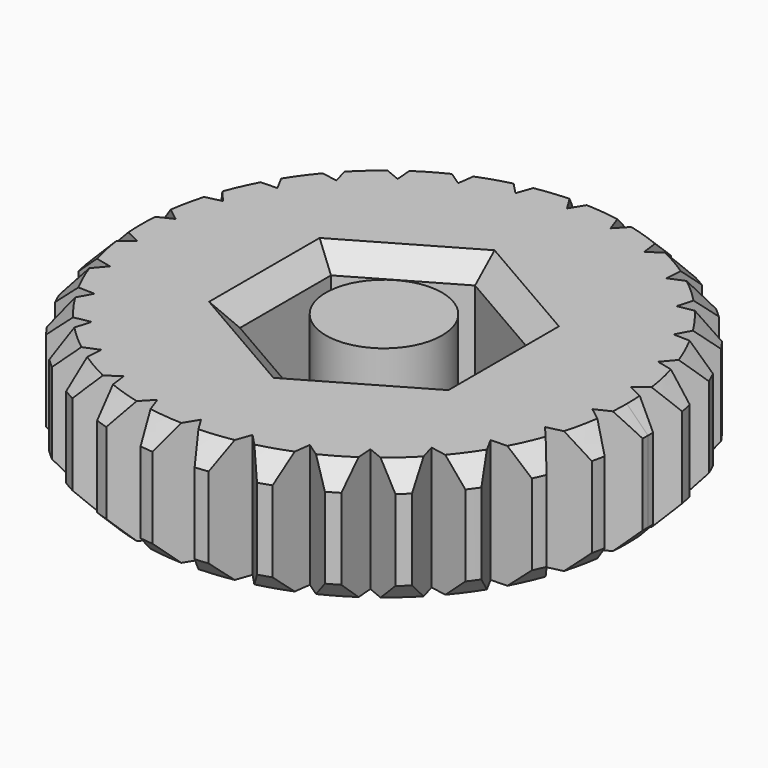
from build123d import *

# Parameters (mm, degrees)
F0_R            = 4
F1_DEPTH        = 5
F2_DEPTH        = 1.5
F0_R_2          = 1.65
F3_DEPTH        = 1.5
F4_SIZE         = 0.6
F5_DEPTH        = 5
F5_COPIES_COUNT = 30
F6_R            = 1.65
F7_DEPTH        = 3.5


# Not quite as in the source:
# - a pattern or mirror of a feature is missing from the dataset's text; its kind, count and spacing are read off the source's solid


with BuildPart() as f1:
    # F0 (on Top) → F1 (new body)
    with BuildSketch(Plane.XY):
        with BuildLine():
            ThreePointArc((-0.6, 7.4759614766), (-5.0867474873, -5.5113519213), (7.5, 0))
            ThreePointArc((7.5, 0), (5.5113519213, 5.0867474873), (0.6, 7.4759614766))
            Line((0.6, 7.4759614766), (0, 6.5))
            Line((0, 6.5), (-0.6, 7.4759614766))
        make_face()
        Circle(F0_R, mode=Mode.SUBTRACT)
        Circle(F0_R)
        Polygon((0, -3.2331615075), (-2.8, -1.6165807537), (-2.8, 1.6165807537), (0, 3.2331615075), (2.8, 1.6165807537), (2.8, -1.6165807537), align=None, mode=Mode.SUBTRACT)
        with BuildLine():
            Line((0, 6.5), (0.6, 7.4759614766))
            ThreePointArc((0.6, 7.4759614766), (0, 7.5), (-0.6, 7.4759614766))
            Line((-0.6, 7.4759614766), (0, 6.5))
        make_face()
    extrude(amount=F1_DEPTH)

    # F0 (on Top) → F2 (cut)
    with BuildSketch(Plane.XY):
        with BuildLine():
            ThreePointArc((-0.6, 7.4759614766), (-5.0867474873, -5.5113519213), (7.5, 0))
            ThreePointArc((7.5, 0), (5.5113519213, 5.0867474873), (0.6, 7.4759614766))
            Line((0.6, 7.4759614766), (0, 6.5))
            Line((0, 6.5), (-0.6, 7.4759614766))
        make_face()
        Circle(F0_R, mode=Mode.SUBTRACT)
        with BuildLine():
            Line((0, 6.5), (0.6, 7.4759614766))
            ThreePointArc((0.6, 7.4759614766), (0, 7.5), (-0.6, 7.4759614766))
            Line((-0.6, 7.4759614766), (0, 6.5))
        make_face()
    extrude(amount=F2_DEPTH, mode=Mode.SUBTRACT)

    # F0 (on Top) → F3 (join)
    with BuildSketch(Plane.XY):
        Polygon((-2.8, 1.6165807537), (-2.8, -1.6165807537), (0, -3.2331615075), (2.8, -1.6165807537), (2.8, 1.6165807537), (0, 3.2331615075), align=None)
        Circle(F0_R_2, mode=Mode.SUBTRACT)
    extrude(amount=F3_DEPTH)

    # F4
    f4_edges = [f1.edges().sort_by_distance(p)[0] for p in [
        (0.6, -7.475961, 1.5),
        (0.6, -7.475961, 5),
        (-4, 0, 1.5),
        (-4, 0, 0),
        (-1.4, 2.424871, 5),
        (-2.8, 0, 5),
        (-1.4, -2.424871, 5),
        (1.4, -2.424871, 5),
        (2.8, 0, 5),
        (1.4, 2.424871, 5),
    ]]
    chamfer(f4_edges, length=F4_SIZE)

    # F0 (on Top) → F5 (cut, through all)
    with BuildSketch(Plane.XY):
        with BuildLine():
            Line((0, 6.5), (0.6, 7.4759614766))
            ThreePointArc((0.6, 7.4759614766), (0, 7.5), (-0.6, 7.4759614766))
            Line((-0.6, 7.4759614766), (0, 6.5))
        make_face()
    f5 = extrude(amount=F5_DEPTH, mode=Mode.SUBTRACT)

    # F5_copies: F5 ×30 about axis
    f5_copies_axis = Axis((0, 0, 0), (0, 0, 1))
    for i in range(1, F5_COPIES_COUNT):
        add(f5.rotate(f5_copies_axis, i * 360 / F5_COPIES_COUNT), mode=Mode.SUBTRACT)


with BuildPart() as f7:
    # F6 (on face) → F7 (new body, through all)
    with BuildSketch(Plane.XY.offset(1.5)):
        Circle(F6_R)
    extrude(amount=F7_DEPTH)


solid = Compound([f1.part, f7.part])
